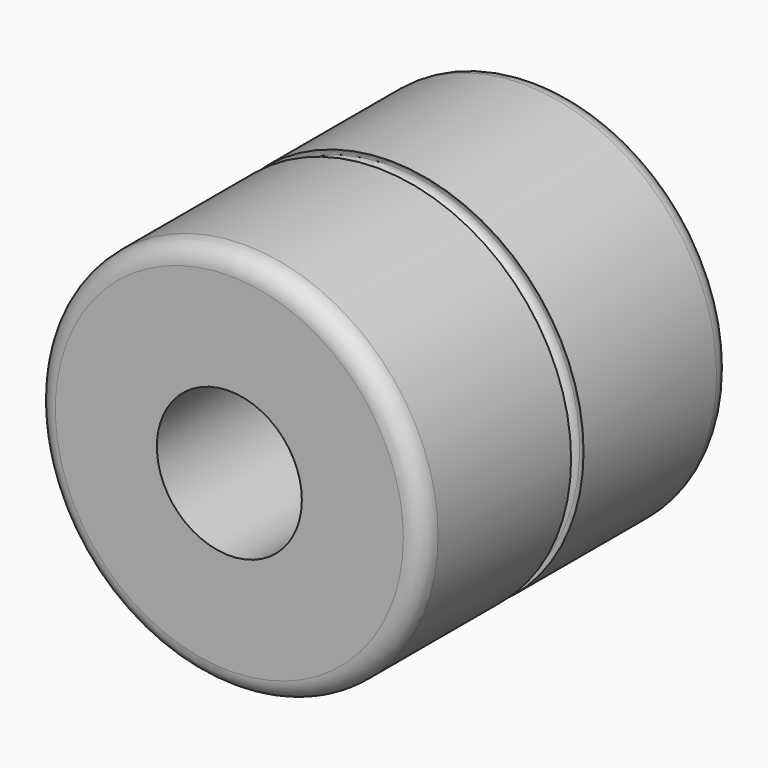
from build123d import *

# Parameters (mm, degrees)
F0_R     = 12.7
F0_R_2   = 4.7625
F1_DEPTH = 12.7
F3_R     = 1.27
F6_R     = 0.6168431606


with BuildPart() as f1:
    # F0 (on Front) → F1 (new body, symmetric)
    with BuildSketch(Plane.XZ):
        Circle(F0_R)
        Circle(F0_R_2, mode=Mode.SUBTRACT)
    extrude(amount=F1_DEPTH, both=True)

    # F3
    f3_edges = [f1.edges().sort_by_distance(p)[0] for p in [
        (-12.7, 12.7, 0),
        (-12.7, -12.7, 0),
    ]]
    fillet(f3_edges, radius=F3_R)

    # F7: sweep along a path in F4
    with BuildLine(Plane(origin=(0, 0, 0), x_dir=(-1, 0, 0), z_dir=(0, 1, 0))) as f7_path:
        CenterArc((0, 0), 12.319, 0, 360)
    # F6 (on line) → F7 (sweep, cut)
    with BuildSketch(Plane.YZ):
        with Locations((0, 12.3572489247)):
            Circle(F6_R)
    sweep(path=f7_path.line, mode=Mode.SUBTRACT)


solid = f1.part
